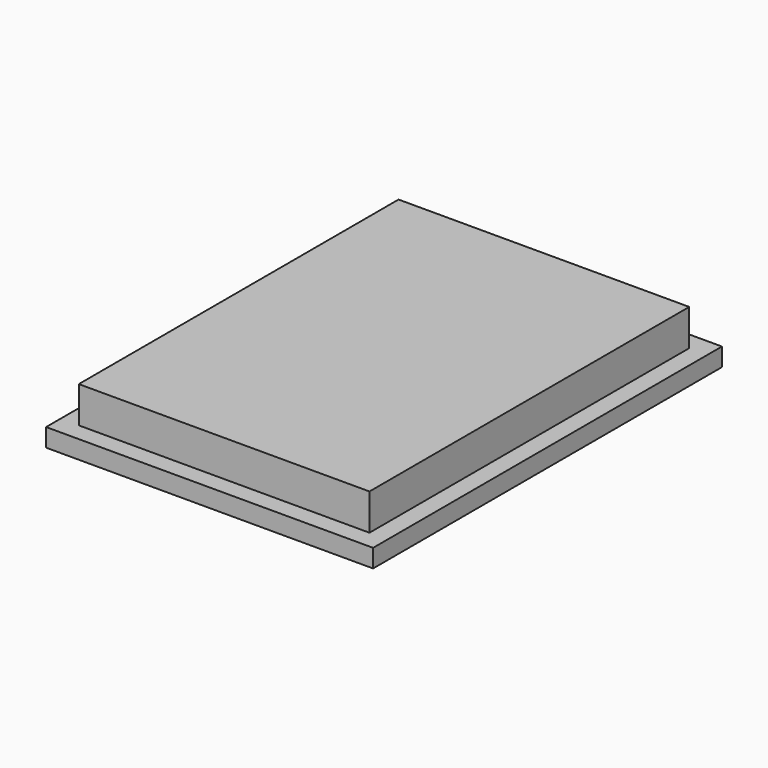
from build123d import *

# Parameters (mm, degrees)
F0_W     = 900
F0_H     = 1200
F1_DEPTH = 50
F3_DEPTH = 100


# Not quite as in the source:
# - the program builds the solid bodies; features that only make, move or delete a surface that nothing else refers to are left out


with BuildPart() as f1:
    # F0 (on Top) → F1 (new body)
    with BuildSketch(Plane.XY):
        Rectangle(F0_W, F0_H)
    extrude(amount=-F1_DEPTH)

    # F2 (on face) → F3 (join)
    with BuildSketch(Plane.XY):
        with BuildLine():
            Line((-400.0000059605, -525), (-400.0000059605, -550))
            Line((-400.0000059605, -550), (-375.0000059605, -550))
            ThreePointArc((-375.0000059605, -550), (-382.3223364308, -532.3223304703), (-400.0000059605, -525))
        make_face()
        with BuildLine():
            ThreePointArc((-400.0000059605, -525), (-382.3223364308, -532.3223304703), (-375.0000059605, -550))
            Line((-375.0000059605, -550), (375, -550))
            ThreePointArc((375, -550), (382.3223304703, -532.3223304703), (400, -525))
            Line((400, -525), (400, 550))
            Line((400, 550), (-400.0000059605, 550))
            Line((-400.0000059605, 550), (-400.0000059605, -525))
        make_face()
        with BuildLine():
            ThreePointArc((400, -525), (382.3223304703, -532.3223304703), (375, -550))
            Line((375, -550), (400, -550))
            Line((400, -550), (400, -525))
        make_face()
    extrude(amount=F3_DEPTH)


solid = f1.part
